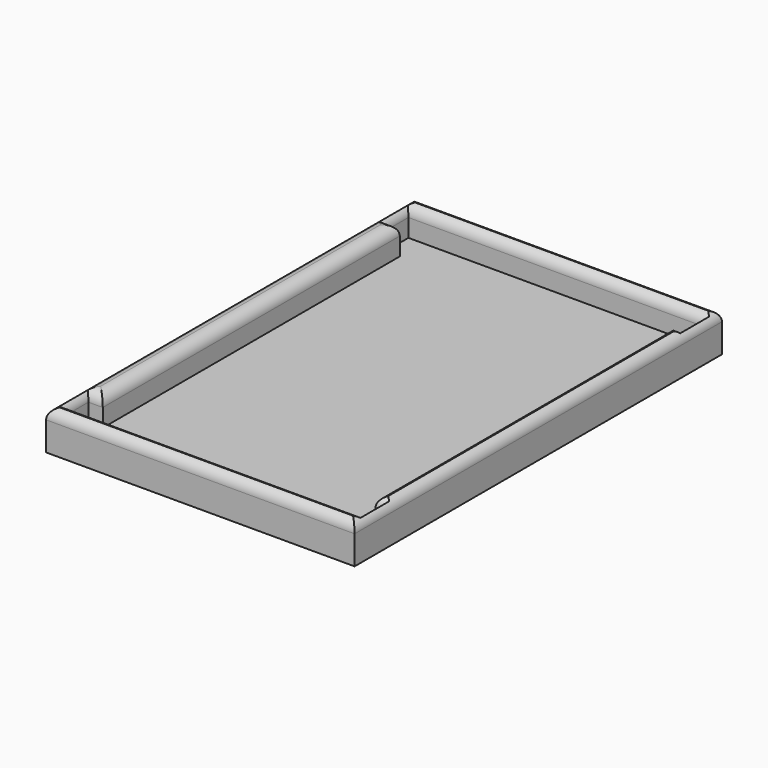
from build123d import *

# Parameters (mm, degrees)
F1_W          = 86
F1_H          = 128
F2_DEPTH      = 8
F0_W          = 86
F0_H          = 128
F3_DEPTH      = 3
F4_T1_DEPTH   = 118.5
F4_T3_DEPTH   = 101
F4_T5_DEPTH   = 143
F4_T7_DEPTH   = 8
F4_T9_DEPTH   = 82
F4_T11_DEPTH  = 9.5
F4_T13_DEPTH  = 8
F4_T15_DEPTH  = 11.5
F4_T21_DEPTH  = 15.5
F4_T26_DEPTH  = 11.5
F4_T34_DEPTH  = 15.5
F4_T40_DEPTH  = 89.5
F4_T48_DEPTH  = 89.5
F4_T53_DEPTH  = 15.5
F4_T62_DEPTH  = 15.5
F4_T67_DEPTH  = 9.5
F4_T75_DEPTH  = 9.5
F4_T80_DEPTH  = 15.5
F4_T88_DEPTH  = 15.5
F4_T94_DEPTH  = 89.5
F4_T102_DEPTH = 89.5
F4_T107_DEPTH = 15.5
F4_T116_DEPTH = 15.5
F4_T121_DEPTH = 11.5


# Not quite as in the source:
# - a fillet or chamfer that OpenCascade refuses, or shapes differently, is made with other operations: its cross-section is extruded or revolved along the edge and cut away or added


with BuildPart() as f2:
    # F1 (on face) → F2 (new body)
    with BuildSketch(Plane.XY):
        Rectangle(F1_W, F1_H)
        Polygon((-41, 51.75), (-41, 59.75), (41, 59.75), (41, 51.75), (39, 51.75), (39, -51.75), (41, -51.75), (41, -59.75), (-41, -59.75), (-41, -51.75), (-37, -51.75), (-37, 51.75), align=None, mode=Mode.SUBTRACT)
    extrude(amount=F2_DEPTH)

    # F0 (on Top) → F3 (join)
    with BuildSketch(Plane.XY):
        Rectangle(F0_W, F0_H)
    extrude(amount=-F3_DEPTH)

    # F4: fillet of radius 3 on 16 edges, made by hand

    # F4_s2 → F4_t1 (cut)
    with BuildSketch(Plane.XZ.offset(-59.25)):
        with BuildLine():
            ThreePointArc((-40, 8), (-37.8786796564, 7.1213203436), (-37, 5))
            Line((-37, 5), (-37, 8))
            Line((-37, 8), (-40, 8))
        make_face()
        with BuildLine():
            ThreePointArc((42, 8), (39.8786796564, 7.1213203436), (39, 5))
            Line((39, 5), (39, 8))
            Line((39, 8), (42, 8))
        make_face()
    extrude(amount=F4_T1_DEPTH, mode=Mode.SUBTRACT)

    # F4_s4 → F4_t3 (cut)
    with BuildSketch(Plane.YZ.offset(-50.5)):
        with BuildLine():
            ThreePointArc((64, 5), (63.1213203436, 7.1213203436), (61, 8))
            Line((61, 8), (64, 8))
            Line((64, 8), (64, 5))
        make_face()
        with BuildLine():
            ThreePointArc((-64, 5), (-63.1213203436, 7.1213203436), (-61, 8))
            Line((-61, 8), (-64, 8))
            Line((-64, 8), (-64, 5))
        make_face()
    extrude(amount=F4_T3_DEPTH, mode=Mode.SUBTRACT)

    # F4_s6 → F4_t5 (cut)
    with BuildSketch(Plane.XZ.offset(-71.5)):
        with BuildLine():
            ThreePointArc((-43, 5), (-42.1213203436, 7.1213203436), (-40, 8))
            Line((-40, 8), (-43, 8))
            Line((-43, 8), (-43, 5))
        make_face()
        with BuildLine():
            ThreePointArc((40, 8), (42.1213203436, 7.1213203436), (43, 5))
            Line((43, 5), (43, 8))
            Line((43, 8), (40, 8))
        make_face()
    extrude(amount=F4_T5_DEPTH, mode=Mode.SUBTRACT)

    # F4_s8 → F4_t7 (cut)
    with BuildSketch(Plane.XZ.offset(-59.75)):
        with BuildLine():
            ThreePointArc((-44, 8), (-41.8786796564, 7.1213203436), (-41, 5))
            Line((-41, 5), (-41, 8))
            Line((-41, 8), (-44, 8))
        make_face()
        with BuildLine():
            ThreePointArc((44, 8), (41.8786796564, 7.1213203436), (41, 5))
            Line((41, 5), (41, 8))
            Line((41, 8), (44, 8))
        make_face()
    extrude(amount=F4_T7_DEPTH, mode=Mode.SUBTRACT)

    # F4_s10 → F4_t9 (cut)
    with BuildSketch(Plane.YZ.offset(-41)):
        with BuildLine():
            ThreePointArc((62.75, 8), (60.6286796564, 7.1213203436), (59.75, 5))
            Line((59.75, 5), (59.75, 8))
            Line((59.75, 8), (62.75, 8))
        make_face()
        with BuildLine():
            ThreePointArc((-62.75, 8), (-60.6286796564, 7.1213203436), (-59.75, 5))
            Line((-59.75, 5), (-59.75, 8))
            Line((-59.75, 8), (-62.75, 8))
        make_face()
    extrude(amount=F4_T9_DEPTH, mode=Mode.SUBTRACT)

    # F4_s12 → F4_t11 (cut)
    with BuildSketch(Plane.YZ.offset(31.5)):
        with BuildLine():
            ThreePointArc((48.75, 8), (50.8713203436, 7.1213203436), (51.75, 5))
            Line((51.75, 5), (51.75, 8))
            Line((51.75, 8), (48.75, 8))
        make_face()
        with BuildLine():
            ThreePointArc((-48.75, 8), (-50.8713203436, 7.1213203436), (-51.75, 5))
            Line((-51.75, 5), (-51.75, 8))
            Line((-51.75, 8), (-48.75, 8))
        make_face()
    extrude(amount=F4_T11_DEPTH, mode=Mode.SUBTRACT)

    # F4_s14 → F4_t13 (cut)
    with BuildSketch(Plane.XZ.offset(51.75)):
        with BuildLine():
            ThreePointArc((44, 8), (41.8786796564, 7.1213203436), (41, 5))
            Line((41, 5), (41, 8))
            Line((41, 8), (44, 8))
        make_face()
        with BuildLine():
            ThreePointArc((-44, 8), (-41.8786796564, 7.1213203436), (-41, 5))
            Line((-41, 5), (-41, 8))
            Line((-41, 8), (-44, 8))
        make_face()
    extrude(amount=F4_T13_DEPTH, mode=Mode.SUBTRACT)

    # F4_s16 → F4_t15 (cut)
    with BuildSketch(Plane.YZ.offset(-41)):
        with BuildLine():
            ThreePointArc((-48.75, 8), (-50.8713203436, 7.1213203436), (-51.75, 5))
            Line((-51.75, 5), (-51.75, 8))
            Line((-51.75, 8), (-48.75, 8))
        make_face()
        with BuildLine():
            ThreePointArc((48.75, 8), (50.8713203436, 7.1213203436), (51.75, 5))
            Line((51.75, 5), (51.75, 8))
            Line((51.75, 8), (48.75, 8))
        make_face()
    extrude(amount=F4_T15_DEPTH, mode=Mode.SUBTRACT)


with BuildPart() as f4_tool19:
    # F4_s20 → F4_t21 (new body)
    with BuildSketch(Plane.XZ.offset(-44.25)):
        with BuildLine():
            ThreePointArc((-44, 8), (-41.8786796564, 7.1213203436), (-41, 5))
            Line((-41, 5), (-41, 8))
            Line((-41, 8), (-44, 8))
        make_face()
    extrude(amount=-F4_T21_DEPTH)

    split(bisect_by=Plane.YZ.offset(-43), keep=Keep.TOP)

    split(bisect_by=Plane.XZ.offset(-51.75), keep=Keep.TOP)


with BuildPart() as f4_tool24:
    # F4_s25 → F4_t26 (new body)
    with BuildSketch(Plane.YZ.offset(-37)):
        with BuildLine():
            ThreePointArc((48.75, 8), (50.8713203436, 7.1213203436), (51.75, 5))
            Line((51.75, 5), (51.75, 8))
            Line((51.75, 8), (48.75, 8))
        make_face()
    extrude(amount=-F4_T26_DEPTH)

    split(bisect_by=Plane.YZ.offset(-43), keep=Keep.TOP)

    split(bisect_by=Plane.YZ.offset(-41), keep=Keep.BOTTOM)


with BuildPart() as f4_tool19_1:
    add(f4_tool19.part)

    # F4_t29: intersect F4_tool24
    add(f4_tool24.part, mode=Mode.INTERSECT)


with BuildPart() as f2_1:
    add(f2.part)

    # F4_t17: cut F4_tool19
    add(f4_tool19_1.part, mode=Mode.SUBTRACT)


with BuildPart() as f4_tool32:
    # F4_s33 → F4_t34 (new body)
    with BuildSketch(Plane.XZ.offset(-51.75)):
        with BuildLine():
            ThreePointArc((-44, 8), (-41.8786796564, 7.1213203436), (-41, 5))
            Line((-41, 5), (-41, 8))
            Line((-41, 8), (-44, 8))
        make_face()
    extrude(amount=-F4_T34_DEPTH)

    split(bisect_by=Plane.XZ.offset(-64), keep=Keep.TOP)

    split(bisect_by=Plane.YZ.offset(-43), keep=Keep.TOP)

    split(bisect_by=Plane.XZ.offset(-59.75), keep=Keep.BOTTOM)


with BuildPart() as f4_tool38:
    # F4_s39 → F4_t40 (new body)
    with BuildSketch(Plane.YZ.offset(-48.5)):
        with BuildLine():
            ThreePointArc((62.75, 8), (60.6286796564, 7.1213203436), (59.75, 5))
            Line((59.75, 5), (59.75, 8))
            Line((59.75, 8), (62.75, 8))
        make_face()
    extrude(amount=F4_T40_DEPTH)

    split(bisect_by=Plane.YZ.offset(-43), keep=Keep.TOP)

    split(bisect_by=Plane.YZ.offset(-41), keep=Keep.BOTTOM)


with BuildPart() as f4_tool32_1:
    add(f4_tool32.part)

    # F4_t43: intersect F4_tool38
    add(f4_tool38.part, mode=Mode.INTERSECT)


with BuildPart() as f2_2:
    add(f2_1.part)

    # F4_t30: cut F4_tool32
    add(f4_tool32_1.part, mode=Mode.SUBTRACT)


with BuildPart() as f4_tool46:
    # F4_s47 → F4_t48 (new body)
    with BuildSketch(Plane.YZ.offset(-41)):
        with BuildLine():
            ThreePointArc((62.75, 8), (60.6286796564, 7.1213203436), (59.75, 5))
            Line((59.75, 5), (59.75, 8))
            Line((59.75, 8), (62.75, 8))
        make_face()
    extrude(amount=F4_T48_DEPTH)

    split(bisect_by=Plane.YZ.offset(41), keep=Keep.TOP)

    split(bisect_by=Plane.YZ.offset(43), keep=Keep.BOTTOM)


with BuildPart() as f4_tool51:
    # F4_s52 → F4_t53 (new body)
    with BuildSketch(Plane.XZ.offset(-67.25)):
        with BuildLine():
            ThreePointArc((44, 8), (41.8786796564, 7.1213203436), (41, 5))
            Line((41, 5), (41, 8))
            Line((41, 8), (44, 8))
        make_face()
    extrude(amount=F4_T53_DEPTH)

    split(bisect_by=Plane.XZ.offset(-64), keep=Keep.TOP)

    split(bisect_by=Plane.XZ.offset(-59.75), keep=Keep.BOTTOM)

    split(bisect_by=Plane.YZ.offset(43), keep=Keep.BOTTOM)


with BuildPart() as f4_tool46_1:
    add(f4_tool46.part)

    # F4_t57: intersect F4_tool51
    add(f4_tool51.part, mode=Mode.INTERSECT)


with BuildPart() as f2_3:
    add(f2_2.part)

    # F4_t44: cut F4_tool46
    add(f4_tool46_1.part, mode=Mode.SUBTRACT)


with BuildPart() as f4_tool60:
    # F4_s61 → F4_t62 (new body)
    with BuildSketch(Plane.XZ.offset(-59.75)):
        with BuildLine():
            ThreePointArc((44, 8), (41.8786796564, 7.1213203436), (41, 5))
            Line((41, 5), (41, 8))
            Line((41, 8), (44, 8))
        make_face()
    extrude(amount=F4_T62_DEPTH)

    split(bisect_by=Plane.XZ.offset(-51.75), keep=Keep.TOP)

    split(bisect_by=Plane.YZ.offset(43), keep=Keep.BOTTOM)


with BuildPart() as f4_tool65:
    # F4_s66 → F4_t67 (new body)
    with BuildSketch(Plane.YZ.offset(48.5)):
        with BuildLine():
            ThreePointArc((48.75, 8), (50.8713203436, 7.1213203436), (51.75, 5))
            Line((51.75, 5), (51.75, 8))
            Line((51.75, 8), (48.75, 8))
        make_face()
    extrude(amount=-F4_T67_DEPTH)

    split(bisect_by=Plane.YZ.offset(41), keep=Keep.TOP)

    split(bisect_by=Plane.YZ.offset(43), keep=Keep.BOTTOM)


with BuildPart() as f4_tool60_1:
    add(f4_tool60.part)

    # F4_t70: intersect F4_tool65
    add(f4_tool65.part, mode=Mode.INTERSECT)


with BuildPart() as f2_4:
    add(f2_3.part)

    # F4_t58: cut F4_tool60
    add(f4_tool60_1.part, mode=Mode.SUBTRACT)


with BuildPart() as f4_tool73:
    # F4_s74 → F4_t75 (new body)
    with BuildSketch(Plane.YZ.offset(39)):
        with BuildLine():
            ThreePointArc((-48.75, 8), (-50.8713203436, 7.1213203436), (-51.75, 5))
            Line((-51.75, 5), (-51.75, 8))
            Line((-51.75, 8), (-48.75, 8))
        make_face()
    extrude(amount=F4_T75_DEPTH)

    split(bisect_by=Plane.YZ.offset(41), keep=Keep.TOP)

    split(bisect_by=Plane.YZ.offset(43), keep=Keep.BOTTOM)


with BuildPart() as f4_tool78:
    # F4_s79 → F4_t80 (new body)
    with BuildSketch(Plane.XZ.offset(44.25)):
        with BuildLine():
            ThreePointArc((44, 8), (41.8786796564, 7.1213203436), (41, 5))
            Line((41, 5), (41, 8))
            Line((41, 8), (44, 8))
        make_face()
    extrude(amount=F4_T80_DEPTH)

    split(bisect_by=Plane.XZ.offset(51.75), keep=Keep.BOTTOM)

    split(bisect_by=Plane.YZ.offset(43), keep=Keep.BOTTOM)


with BuildPart() as f4_tool73_1:
    add(f4_tool73.part)

    # F4_t83: intersect F4_tool78
    add(f4_tool78.part, mode=Mode.INTERSECT)


with BuildPart() as f2_5:
    add(f2_4.part)

    # F4_t71: cut F4_tool73
    add(f4_tool73_1.part, mode=Mode.SUBTRACT)


with BuildPart() as f4_tool86:
    # F4_s87 → F4_t88 (new body)
    with BuildSketch(Plane.XZ.offset(51.75)):
        with BuildLine():
            ThreePointArc((44, 8), (41.8786796564, 7.1213203436), (41, 5))
            Line((41, 5), (41, 8))
            Line((41, 8), (44, 8))
        make_face()
    extrude(amount=F4_T88_DEPTH)

    split(bisect_by=Plane.XZ.offset(64), keep=Keep.BOTTOM)

    split(bisect_by=Plane.XZ.offset(59.75), keep=Keep.TOP)

    split(bisect_by=Plane.YZ.offset(43), keep=Keep.BOTTOM)


with BuildPart() as f4_tool92:
    # F4_s93 → F4_t94 (new body)
    with BuildSketch(Plane.YZ.offset(48.5)):
        with BuildLine():
            ThreePointArc((-62.75, 8), (-60.6286796564, 7.1213203436), (-59.75, 5))
            Line((-59.75, 5), (-59.75, 8))
            Line((-59.75, 8), (-62.75, 8))
        make_face()
    extrude(amount=-F4_T94_DEPTH)

    split(bisect_by=Plane.YZ.offset(41), keep=Keep.TOP)

    split(bisect_by=Plane.YZ.offset(43), keep=Keep.BOTTOM)


with BuildPart() as f4_tool86_1:
    add(f4_tool86.part)

    # F4_t97: intersect F4_tool92
    add(f4_tool92.part, mode=Mode.INTERSECT)


with BuildPart() as f2_6:
    add(f2_5.part)

    # F4_t84: cut F4_tool86
    add(f4_tool86_1.part, mode=Mode.SUBTRACT)


with BuildPart() as f4_tool100:
    # F4_s101 → F4_t102 (new body)
    with BuildSketch(Plane.YZ.offset(41)):
        with BuildLine():
            ThreePointArc((-62.75, 8), (-60.6286796564, 7.1213203436), (-59.75, 5))
            Line((-59.75, 5), (-59.75, 8))
            Line((-59.75, 8), (-62.75, 8))
        make_face()
    extrude(amount=-F4_T102_DEPTH)

    split(bisect_by=Plane.YZ.offset(-43), keep=Keep.TOP)

    split(bisect_by=Plane.YZ.offset(-41), keep=Keep.BOTTOM)


with BuildPart() as f4_tool105:
    # F4_s106 → F4_t107 (new body)
    with BuildSketch(Plane.XZ.offset(67.25)):
        with BuildLine():
            ThreePointArc((-44, 8), (-41.8786796564, 7.1213203436), (-41, 5))
            Line((-41, 5), (-41, 8))
            Line((-41, 8), (-44, 8))
        make_face()
    extrude(amount=-F4_T107_DEPTH)

    split(bisect_by=Plane.XZ.offset(64), keep=Keep.BOTTOM)

    split(bisect_by=Plane.YZ.offset(-43), keep=Keep.TOP)

    split(bisect_by=Plane.XZ.offset(59.75), keep=Keep.TOP)


with BuildPart() as f4_tool100_1:
    add(f4_tool100.part)

    # F4_t111: intersect F4_tool105
    add(f4_tool105.part, mode=Mode.INTERSECT)


with BuildPart() as f2_7:
    add(f2_6.part)

    # F4_t98: cut F4_tool100
    add(f4_tool100_1.part, mode=Mode.SUBTRACT)


with BuildPart() as f4_tool114:
    # F4_s115 → F4_t116 (new body)
    with BuildSketch(Plane.XZ.offset(59.75)):
        with BuildLine():
            ThreePointArc((-44, 8), (-41.8786796564, 7.1213203436), (-41, 5))
            Line((-41, 5), (-41, 8))
            Line((-41, 8), (-44, 8))
        make_face()
    extrude(amount=-F4_T116_DEPTH)

    split(bisect_by=Plane.YZ.offset(-43), keep=Keep.TOP)

    split(bisect_by=Plane.XZ.offset(51.75), keep=Keep.BOTTOM)


with BuildPart() as f4_tool119:
    # F4_s120 → F4_t121 (new body)
    with BuildSketch(Plane.YZ.offset(-48.5)):
        with BuildLine():
            ThreePointArc((-48.75, 8), (-50.8713203436, 7.1213203436), (-51.75, 5))
            Line((-51.75, 5), (-51.75, 8))
            Line((-51.75, 8), (-48.75, 8))
        make_face()
    extrude(amount=F4_T121_DEPTH)

    split(bisect_by=Plane.YZ.offset(-43), keep=Keep.TOP)

    split(bisect_by=Plane.YZ.offset(-41), keep=Keep.BOTTOM)


with BuildPart() as f4_tool114_1:
    add(f4_tool114.part)

    # F4_t124: intersect F4_tool119
    add(f4_tool119.part, mode=Mode.INTERSECT)


with BuildPart() as f2_8:
    add(f2_7.part)

    # F4_t112: cut F4_tool114
    add(f4_tool114_1.part, mode=Mode.SUBTRACT)


solid = f2_8.part
